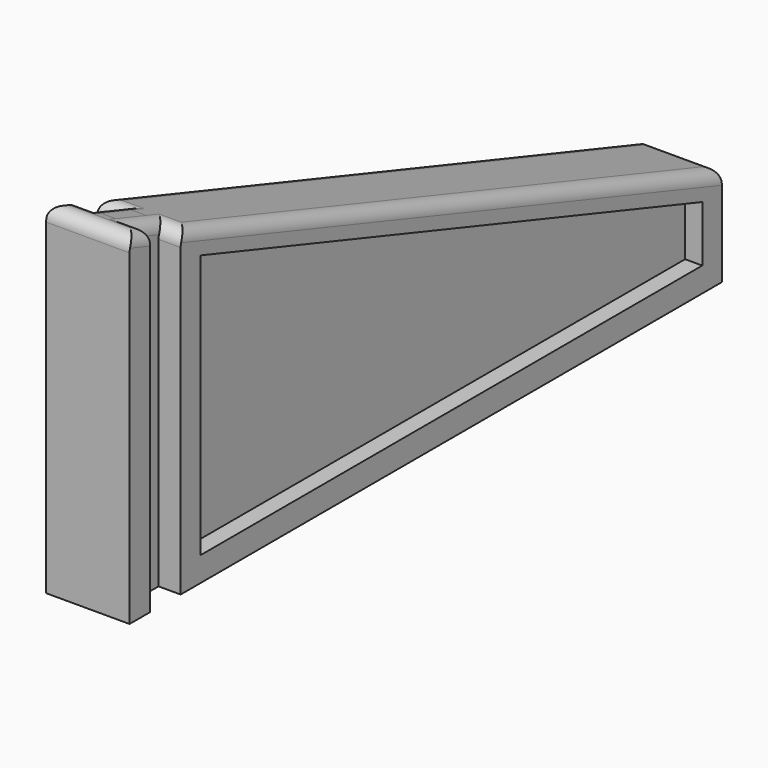
from build123d import *

# Parameters (mm, degrees)
F1_DEPTH     = 1.6
F2_DEPTH     = 3.4
F3_T         = -2
F5_T1_DEPTH  = 10.409799149
F5_T3_DEPTH  = 63.0683209094
F5_T5_DEPTH  = 5.2627965391
F5_T7_DEPTH  = 3.6048995745
F5_T9_DEPTH  = 7.2124323677
F5_T11_DEPTH = 13.7255930783
F5_T13_DEPTH = 3.6048995745
F5_T15_DEPTH = 5.2627965391
F5_T20_DEPTH = 8.7255930783
F5_T25_DEPTH = 8.2659715904
F5_T31_DEPTH = 8.2659715904
F5_T37_DEPTH = 8.7255930783
F5_T43_DEPTH = 8.7255930783
F5_T48_DEPTH = 8.2659715904
F5_T55_DEPTH = 8.2659715904
F5_T59_DEPTH = 5.409799149
F5_T66_DEPTH = 5.409799149
F5_T70_DEPTH = 8.2659715904
F5_T77_DEPTH = 8.2659715904
F5_T81_DEPTH = 8.7255930783


# Not quite as in the source:
# - a fillet or chamfer that OpenCascade refuses, or shapes differently, is made with other operations: its cross-section is extruded or revolved along the edge and cut away or added


with BuildPart() as f1:
    # F0 (on Right) → F1 (new body)
    with BuildSketch(Plane.YZ):
        Polygon((-50.2783237807, 58.1370850594), (-53.3783237807, 59.1649811775), (-53.3783237807, 31.8612979027), (-50.2783237807, 31.8612979027), align=None)
    extrude(amount=F1_DEPTH)

    # F0 (on Right) → F2 (join)
    with BuildSketch(Plane.YZ):
        Polygon((4.8390554843, 39.8612979027), (-50.2783237807, 58.1370850594), (-50.2783237807, 31.8612979027), (4.8390554843, 31.8612979027), align=None)
        Polygon((-53.3783237807, 59.1649811775), (-55.4783237807, 59.8612979027), (-55.4783237807, 31.8612979027), (-53.3783237807, 31.8612979027), align=None)
    extrude(amount=F2_DEPTH)

    # F3
    f3_openings = [f1.faces().sort_by_distance(p)[0] for p in [
        (3.4, -27.617715, 41.242296),
    ]]
    offset(amount=F3_T, openings=f3_openings)

    # F4: F1 across face


with BuildPart() as f1_1:
    add(f1.part)
    add(f1.part.mirror(Plane.YZ))

    # F5: fillet of radius 1 on 12 edges, made by hand

    # F5_s2 → F5_t1 (cut)
    with BuildSketch(Plane.YZ.offset(-5.2048995745)):
        with BuildLine():
            ThreePointArc((4.1537845288, 40.0885196301), (4.6498356778, 39.7246888034), (4.8390554843, 39.1393380729))
            Line((4.8390554843, 39.1393380729), (4.8390554843, 39.8612979027))
            Line((4.8390554843, 39.8612979027), (4.1537845288, 40.0885196301))
        make_face()
    extrude(amount=F5_T1_DEPTH, mode=Mode.SUBTRACT)

    # F5_s4 → F5_t3 (cut)
    with BuildSketch(Plane(origin=(0, -5.1752852335, 1.716017936), x_dir=(1, 0, 0), z_dir=(0, -0.9491815572, 0.3147290445))):
        with BuildLine():
            ThreePointArc((2.4, 39.3586001244), (3.1071067812, 39.0657069056), (3.4, 38.3586001244))
            Line((3.4, 38.3586001244), (3.4, 39.3586001244))
            Line((3.4, 39.3586001244), (2.4, 39.3586001244))
        make_face()
        with BuildLine():
            ThreePointArc((-2.4, 39.3586001244), (-3.1071067812, 39.0657069056), (-3.4, 38.3586001244))
            Line((-3.4, 38.3586001244), (-3.4, 39.3586001244))
            Line((-3.4, 39.3586001244), (-2.4, 39.3586001244))
        make_face()
    extrude(amount=F5_T3_DEPTH, mode=Mode.SUBTRACT)

    # F5_s6 → F5_t5 (cut)
    with BuildSketch(Plane.YZ.offset(1.6)):
        with BuildLine():
            ThreePointArc((-48.9635947362, 57.701148001), (-49.8636745112, 57.5627466373), (-50.2783237807, 56.7519664438))
            Line((-50.2783237807, 56.7519664438), (-50.2783237807, 58.1370850594))
            Line((-50.2783237807, 58.1370850594), (-48.9635947362, 57.701148001))
        make_face()
    extrude(amount=F5_T5_DEPTH, mode=Mode.SUBTRACT)

    # F5_s8 → F5_t7 (cut)
    with BuildSketch(Plane.YZ.offset(1.6)):
        with BuildLine():
            ThreePointArc((-54.0635947362, 59.3922029049), (-53.5675435871, 59.0283720783), (-53.3783237807, 58.4430213477))
            Line((-53.3783237807, 58.4430213477), (-53.3783237807, 59.1649811775))
            Line((-53.3783237807, 59.1649811775), (-54.0635947362, 59.3922029049))
        make_face()
    extrude(amount=F5_T7_DEPTH, mode=Mode.SUBTRACT)

    # F5_s10 → F5_t9 (cut)
    with BuildSketch(Plane(origin=(0, -63.3926644985, 21.0197012108), x_dir=(1, 0, 0), z_dir=(0, -0.9491815572, 0.3147290445))):
        with BuildLine():
            ThreePointArc((2.4, 39.3586001244), (3.1071067812, 39.0657069056), (3.4, 38.3586001244))
            Line((3.4, 38.3586001244), (3.4, 39.3586001244))
            Line((3.4, 39.3586001244), (2.4, 39.3586001244))
        make_face()
        with BuildLine():
            ThreePointArc((-2.4, 39.3586001244), (-3.1071067812, 39.0657069056), (-3.4, 38.3586001244))
            Line((-3.4, 38.3586001244), (-3.4, 39.3586001244))
            Line((-3.4, 39.3586001244), (-2.4, 39.3586001244))
        make_face()
    extrude(amount=F5_T9_DEPTH, mode=Mode.SUBTRACT)

    # F5_s12 → F5_t11 (cut)
    with BuildSketch(Plane.YZ.offset(-6.8627965391)):
        with BuildLine():
            ThreePointArc((-54.1635947362, 59.4253608442), (-55.0636745112, 59.2869594806), (-55.4783237807, 58.476179287))
            Line((-55.4783237807, 58.476179287), (-55.4783237807, 59.8612979027))
            Line((-55.4783237807, 59.8612979027), (-54.1635947362, 59.4253608442))
        make_face()
    extrude(amount=F5_T11_DEPTH, mode=Mode.SUBTRACT)

    # F5_s14 → F5_t13 (cut)
    with BuildSketch(Plane.YZ.offset(-5.2048995745)):
        with BuildLine():
            ThreePointArc((-54.0635947362, 59.3922029049), (-53.5675435871, 59.0283720783), (-53.3783237807, 58.4430213477))
            Line((-53.3783237807, 58.4430213477), (-53.3783237807, 59.1649811775))
            Line((-53.3783237807, 59.1649811775), (-54.0635947362, 59.3922029049))
        make_face()
    extrude(amount=F5_T13_DEPTH, mode=Mode.SUBTRACT)

    # F5_s16 → F5_t15 (cut)
    with BuildSketch(Plane.YZ.offset(-6.8627965391)):
        with BuildLine():
            ThreePointArc((-48.9635947362, 57.701148001), (-49.8636745112, 57.5627466373), (-50.2783237807, 56.7519664438))
            Line((-50.2783237807, 56.7519664438), (-50.2783237807, 58.1370850594))
            Line((-50.2783237807, 58.1370850594), (-48.9635947362, 57.701148001))
        make_face()
    extrude(amount=F5_T15_DEPTH, mode=Mode.SUBTRACT)


with BuildPart() as f5_tool18:
    # F5_s19 → F5_t20 (new body)
    with BuildSketch(Plane.YZ.offset(-1.8627965391)):
        with BuildLine():
            ThreePointArc((-48.9635947362, 57.701148001), (-49.8636745112, 57.5627466373), (-50.2783237807, 56.7519664438))
            Line((-50.2783237807, 56.7519664438), (-50.2783237807, 58.1370850594))
            Line((-50.2783237807, 58.1370850594), (-48.9635947362, 57.701148001))
        make_face()
    extrude(amount=F5_T20_DEPTH)

    split(bisect_by=Plane.YZ.offset(-1.6), keep=Keep.BOTTOM)


with BuildPart() as f1_2:
    add(f1_1.part)

    # F5_t17: cut F5_tool18
    add(f5_tool18.part, mode=Mode.SUBTRACT)


with BuildPart() as f5_tool23:
    # F5_s24 → F5_t25 (new body)
    with BuildSketch(Plane(origin=(0, -60.2926644985, 19.9918050927), x_dir=(1, 0, 0), z_dir=(0, -0.9491815572, 0.3147290445))):
        with BuildLine():
            ThreePointArc((0.6, 39.3586001244), (1.3071067812, 39.0657069056), (1.6, 38.3586001244))
            Line((1.6, 38.3586001244), (1.6, 39.3586001244))
            Line((1.6, 39.3586001244), (0.6, 39.3586001244))
        make_face()
    extrude(amount=F5_T25_DEPTH)

    split(bisect_by=Plane.XZ.offset(53.3783237807), keep=Keep.BOTTOM)

    split(bisect_by=Plane.XZ.offset(50.2783237807), keep=Keep.TOP)


with BuildPart() as f1_3:
    add(f1_2.part)

    # F5_t22: cut F5_tool23
    add(f5_tool23.part, mode=Mode.SUBTRACT)


with BuildPart() as f5_tool29:
    # F5_s30 → F5_t31 (new body)
    with BuildSketch(Plane(origin=(0, -60.2926644985, 19.9918050927), x_dir=(1, 0, 0), z_dir=(0, -0.9491815572, 0.3147290445))):
        with BuildLine():
            ThreePointArc((-0.6, 39.3586001244), (-1.3071067812, 39.0657069056), (-1.6, 38.3586001244))
            Line((-1.6, 38.3586001244), (-1.6, 39.3586001244))
            Line((-1.6, 39.3586001244), (-0.6, 39.3586001244))
        make_face()
    extrude(amount=F5_T31_DEPTH)

    split(bisect_by=Plane.XZ.offset(50.2783237807), keep=Keep.TOP)

    split(bisect_by=Plane.XZ.offset(53.3783237807), keep=Keep.BOTTOM)


with BuildPart() as f1_4:
    add(f1_3.part)

    # F5_t28: cut F5_tool29
    add(f5_tool29.part, mode=Mode.SUBTRACT)


with BuildPart() as f5_tool35:
    # F5_s36 → F5_t37 (new body)
    with BuildSketch(Plane.YZ.offset(1.8627965391)):
        with BuildLine():
            ThreePointArc((-48.9635947362, 57.701148001), (-49.8636745112, 57.5627466373), (-50.2783237807, 56.7519664438))
            Line((-50.2783237807, 56.7519664438), (-50.2783237807, 58.1370850594))
            Line((-50.2783237807, 58.1370850594), (-48.9635947362, 57.701148001))
        make_face()
    extrude(amount=-F5_T37_DEPTH)

    split(bisect_by=Plane.YZ.offset(1.6), keep=Keep.TOP)


with BuildPart() as f1_5:
    add(f1_4.part)

    # F5_t34: cut F5_tool35
    add(f5_tool35.part, mode=Mode.SUBTRACT)


with BuildPart() as f5_tool41:
    # F5_s42 → F5_t43 (new body)
    with BuildSketch(Plane.YZ.offset(-1.8627965391)):
        with BuildLine():
            ThreePointArc((-48.9635947362, 57.701148001), (-49.8636745112, 57.5627466373), (-50.2783237807, 56.7519664438))
            Line((-50.2783237807, 56.7519664438), (-50.2783237807, 58.1370850594))
            Line((-50.2783237807, 58.1370850594), (-48.9635947362, 57.701148001))
        make_face()
    extrude(amount=F5_T43_DEPTH)

    split(bisect_by=Plane.YZ.offset(-1.6), keep=Keep.TOP)

    split(bisect_by=Plane.YZ.offset(1.6), keep=Keep.BOTTOM)


with BuildPart() as f5_tool46:
    # F5_s47 → F5_t48 (new body)
    with BuildSketch(Plane(origin=(0, -60.2926644985, 19.9918050927), x_dir=(1, 0, 0), z_dir=(0, -0.9491815572, 0.3147290445))):
        with BuildLine():
            ThreePointArc((0.6, 39.3586001244), (1.3071067812, 39.0657069056), (1.6, 38.3586001244))
            Line((1.6, 38.3586001244), (1.6, 39.3586001244))
            Line((1.6, 39.3586001244), (0.6, 39.3586001244))
        make_face()
    extrude(amount=F5_T48_DEPTH)

    split(bisect_by=Plane.XZ.offset(50.2783237807), keep=Keep.BOTTOM)


with BuildPart() as f5_tool41_1:
    add(f5_tool41.part)

    # F5_t50: intersect F5_tool46
    add(f5_tool46.part, mode=Mode.INTERSECT)


with BuildPart() as f1_6:
    add(f1_5.part)

    # F5_t39: cut F5_tool41
    add(f5_tool41_1.part, mode=Mode.SUBTRACT)


with BuildPart() as f5_tool53:
    # F5_s54 → F5_t55 (new body)
    with BuildSketch(Plane(origin=(0, -60.2926644985, 19.9918050927), x_dir=(1, 0, 0), z_dir=(0, -0.9491815572, 0.3147290445))):
        with BuildLine():
            ThreePointArc((0.6, 39.3586001244), (1.3071067812, 39.0657069056), (1.6, 38.3586001244))
            Line((1.6, 38.3586001244), (1.6, 39.3586001244))
            Line((1.6, 39.3586001244), (0.6, 39.3586001244))
        make_face()
    extrude(amount=F5_T55_DEPTH)

    split(bisect_by=Plane.XZ.offset(53.3783237807), keep=Keep.TOP)


with BuildPart() as f5_tool57:
    # F5_s58 → F5_t59 (new body)
    with BuildSketch(Plane.YZ.offset(-0.2048995745)):
        with BuildLine():
            ThreePointArc((-54.0635947362, 59.3922029049), (-53.5675435871, 59.0283720783), (-53.3783237807, 58.4430213477))
            Line((-53.3783237807, 58.4430213477), (-53.3783237807, 59.1649811775))
            Line((-53.3783237807, 59.1649811775), (-54.0635947362, 59.3922029049))
        make_face()
    extrude(amount=F5_T59_DEPTH)

    split(bisect_by=Plane.YZ.offset(1.6), keep=Keep.BOTTOM)


with BuildPart() as f5_tool53_1:
    add(f5_tool53.part)

    # F5_t61: intersect F5_tool57
    add(f5_tool57.part, mode=Mode.INTERSECT)


with BuildPart() as f1_7:
    add(f1_6.part)

    # F5_t51: cut F5_tool53
    add(f5_tool53_1.part, mode=Mode.SUBTRACT)


with BuildPart() as f5_tool64:
    # F5_s65 → F5_t66 (new body)
    with BuildSketch(Plane.YZ.offset(0.2048995745)):
        with BuildLine():
            ThreePointArc((-54.0635947362, 59.3922029049), (-53.5675435871, 59.0283720783), (-53.3783237807, 58.4430213477))
            Line((-53.3783237807, 58.4430213477), (-53.3783237807, 59.1649811775))
            Line((-53.3783237807, 59.1649811775), (-54.0635947362, 59.3922029049))
        make_face()
    extrude(amount=-F5_T66_DEPTH)

    split(bisect_by=Plane.YZ.offset(-1.6), keep=Keep.TOP)


with BuildPart() as f5_tool68:
    # F5_s69 → F5_t70 (new body)
    with BuildSketch(Plane(origin=(0, -60.2926644985, 19.9918050927), x_dir=(1, 0, 0), z_dir=(0, -0.9491815572, 0.3147290445))):
        with BuildLine():
            ThreePointArc((-0.6, 39.3586001244), (-1.3071067812, 39.0657069056), (-1.6, 38.3586001244))
            Line((-1.6, 38.3586001244), (-1.6, 39.3586001244))
            Line((-1.6, 39.3586001244), (-0.6, 39.3586001244))
        make_face()
    extrude(amount=F5_T70_DEPTH)

    split(bisect_by=Plane.XZ.offset(53.3783237807), keep=Keep.TOP)


with BuildPart() as f5_tool64_1:
    add(f5_tool64.part)

    # F5_t72: intersect F5_tool68
    add(f5_tool68.part, mode=Mode.INTERSECT)


with BuildPart() as f1_8:
    add(f1_7.part)

    # F5_t62: cut F5_tool64
    add(f5_tool64_1.part, mode=Mode.SUBTRACT)


with BuildPart() as f5_tool75:
    # F5_s76 → F5_t77 (new body)
    with BuildSketch(Plane(origin=(0, -60.2926644985, 19.9918050927), x_dir=(1, 0, 0), z_dir=(0, -0.9491815572, 0.3147290445))):
        with BuildLine():
            ThreePointArc((-0.6, 39.3586001244), (-1.3071067812, 39.0657069056), (-1.6, 38.3586001244))
            Line((-1.6, 38.3586001244), (-1.6, 39.3586001244))
            Line((-1.6, 39.3586001244), (-0.6, 39.3586001244))
        make_face()
    extrude(amount=F5_T77_DEPTH)

    split(bisect_by=Plane.XZ.offset(50.2783237807), keep=Keep.BOTTOM)


with BuildPart() as f5_tool79:
    # F5_s80 → F5_t81 (new body)
    with BuildSketch(Plane.YZ.offset(1.8627965391)):
        with BuildLine():
            ThreePointArc((-48.9635947362, 57.701148001), (-49.8636745112, 57.5627466373), (-50.2783237807, 56.7519664438))
            Line((-50.2783237807, 56.7519664438), (-50.2783237807, 58.1370850594))
            Line((-50.2783237807, 58.1370850594), (-48.9635947362, 57.701148001))
        make_face()
    extrude(amount=-F5_T81_DEPTH)

    split(bisect_by=Plane.YZ.offset(-1.6), keep=Keep.TOP)

    split(bisect_by=Plane.YZ.offset(1.6), keep=Keep.BOTTOM)


with BuildPart() as f5_tool75_1:
    add(f5_tool75.part)

    # F5_t84: intersect F5_tool79
    add(f5_tool79.part, mode=Mode.INTERSECT)


with BuildPart() as f1_9:
    add(f1_8.part)

    # F5_t73: cut F5_tool75
    add(f5_tool75_1.part, mode=Mode.SUBTRACT)


solid = f1_9.part
